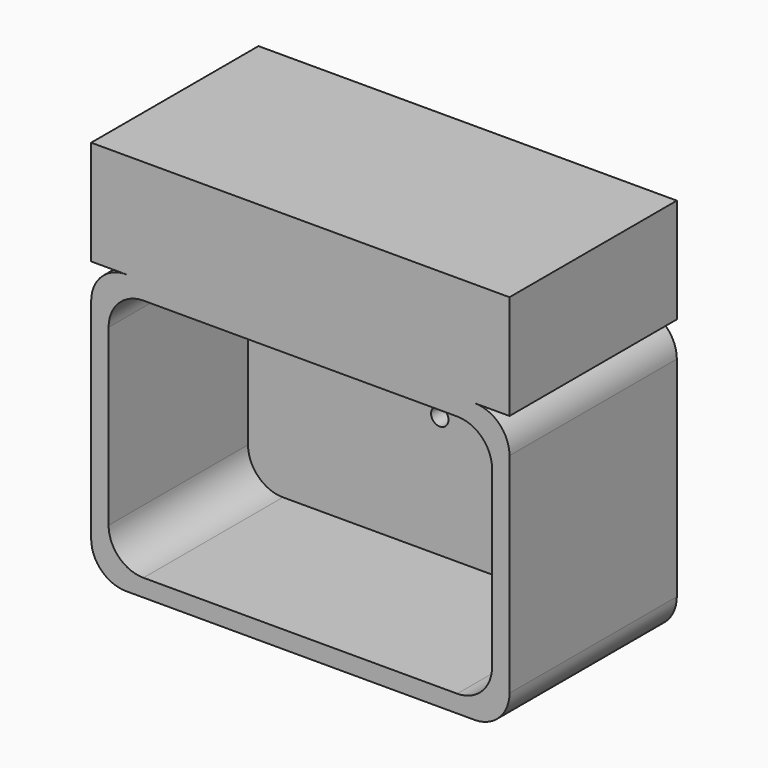
from build123d import *

# Parameters (mm, degrees)
F1_DEPTH = 25.4
F0_R     = 6.35
F2_DEPTH = 152.4
F0_W     = 152.4
F0_H     = 38.1
F3_DEPTH = 152.4


with BuildPart() as f1:
    # F0 (on Front) → F1 (new body)
    with BuildSketch(Plane.XZ):
        Polygon((127, 101.6), (152.4, 101.6), (152.4, 139.7), (0, 139.7), (0, 101.6), align=None)
        Polygon((-127, 101.6), (0, 101.6), (0, 139.7), (-152.4, 139.7), (-152.4, 101.6), align=None)
    extrude(amount=F1_DEPTH)



with BuildPart() as f1b:
    # F0 (on Front) → F1, piece 2 (new body)
    with BuildSketch(Plane.XZ):
        with BuildLine():
            ThreePointArc((139.7, 63.5), (132.2605122421, 81.4605122421), (114.3, 88.9))
            Line((114.3, 88.9), (-114.3, 88.9))
            ThreePointArc((-114.3, 88.9), (-132.2605122421, 81.4605122421), (-139.7, 63.5))
            Line((-139.7, 63.5), (-139.7, -63.5))
            ThreePointArc((-139.7, -63.5), (-132.2605122421, -81.4605122421), (-114.3, -88.9))
            Line((-114.3, -88.9), (114.3, -88.9))
            ThreePointArc((114.3, -88.9), (132.2605122421, -81.4605122421), (139.7, -63.5))
            Line((139.7, -63.5), (139.7, 63.5))
        make_face()
        Circle(F0_R, mode=Mode.SUBTRACT)
    extrude(amount=F1_DEPTH)


with BuildPart() as f1_1:
    add(f1.part)

    add(f1b.part)  # F2 merges F1b
    # F0 (on Front) → F2 (join)
    with BuildSketch(Plane.XZ):
        Polygon((127, 101.6), (152.4, 101.6), (152.4, 139.7), (0, 139.7), (0, 101.6), align=None)
        with BuildLine():
            ThreePointArc((152.4, 76.2), (144.9605122421, 94.1605122421), (127, 101.6))
            Line((127, 101.6), (0, 101.6))
            Line((0, 101.6), (-127, 101.6))
            ThreePointArc((-127, 101.6), (-144.9605122421, 94.1605122421), (-152.4, 76.2))
            Line((-152.4, 76.2), (-152.4, -76.2))
            ThreePointArc((-152.4, -76.2), (-144.9605122421, -94.1605122421), (-127, -101.6))
            Line((-127, -101.6), (127, -101.6))
            ThreePointArc((127, -101.6), (144.9605122421, -94.1605122421), (152.4, -76.2))
            Line((152.4, -76.2), (152.4, 76.2))
        make_face()
        with BuildLine():
            Line((-114.3, 88.9), (114.3, 88.9))
            ThreePointArc((114.3, 88.9), (132.2605122421, 81.4605122421), (139.7, 63.5))
            Line((139.7, 63.5), (139.7, -63.5))
            ThreePointArc((139.7, -63.5), (132.2605122421, -81.4605122421), (114.3, -88.9))
            Line((114.3, -88.9), (-114.3, -88.9))
            ThreePointArc((-114.3, -88.9), (-132.2605122421, -81.4605122421), (-139.7, -63.5))
            Line((-139.7, -63.5), (-139.7, 63.5))
            ThreePointArc((-139.7, 63.5), (-132.2605122421, 81.4605122421), (-114.3, 88.9))
        make_face(mode=Mode.SUBTRACT)
        Polygon((-127, 101.6), (0, 101.6), (0, 139.7), (-152.4, 139.7), (-152.4, 101.6), align=None)
    extrude(amount=F2_DEPTH)

    # F0 (on Front) → F3 (join)
    with BuildSketch(Plane.XZ):
        with BuildLine():
            ThreePointArc((152.4, 76.2), (144.9605122421, 94.1605122421), (127, 101.6))
            Line((127, 101.6), (0, 101.6))
            Line((0, 101.6), (-127, 101.6))
            ThreePointArc((-127, 101.6), (-144.9605122421, 94.1605122421), (-152.4, 76.2))
            Line((-152.4, 76.2), (-152.4, -76.2))
            ThreePointArc((-152.4, -76.2), (-144.9605122421, -94.1605122421), (-127, -101.6))
            Line((-127, -101.6), (127, -101.6))
            ThreePointArc((127, -101.6), (144.9605122421, -94.1605122421), (152.4, -76.2))
            Line((152.4, -76.2), (152.4, 76.2))
        make_face()
        with BuildLine():
            Line((-114.3, 88.9), (114.3, 88.9))
            ThreePointArc((114.3, 88.9), (132.2605122421, 81.4605122421), (139.7, 63.5))
            Line((139.7, 63.5), (139.7, -63.5))
            ThreePointArc((139.7, -63.5), (132.2605122421, -81.4605122421), (114.3, -88.9))
            Line((114.3, -88.9), (-114.3, -88.9))
            ThreePointArc((-114.3, -88.9), (-132.2605122421, -81.4605122421), (-139.7, -63.5))
            Line((-139.7, -63.5), (-139.7, 63.5))
            ThreePointArc((-139.7, 63.5), (-132.2605122421, 81.4605122421), (-114.3, 88.9))
        make_face(mode=Mode.SUBTRACT)
        with Locations((-76.2, 158.75)):
            Rectangle(F0_W, F0_H)
        with Locations((76.2, 158.75)):
            Rectangle(F0_W, F0_H)
    extrude(amount=F3_DEPTH)


solid = f1_1.part
